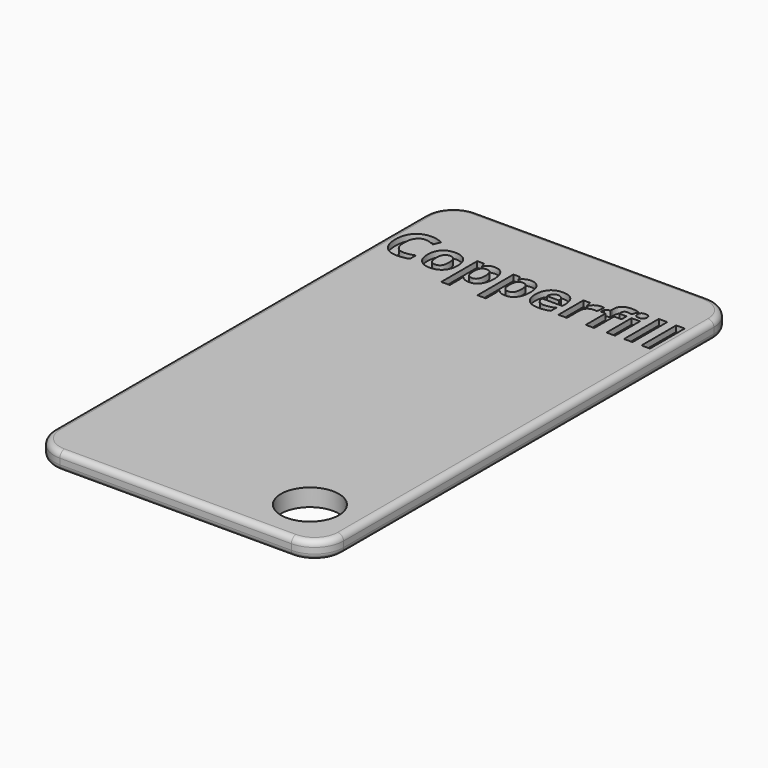
from build123d import *

# Parameters (mm, degrees)
F0_W         = 90
F0_H         = 50
F1_DEPTH     = 3
F2_R         = 1
F3_T1_DEPTH  = 3
F3_T4_ANGLE  = 90
F3_T6_ANGLE  = 90
F3_T8_ANGLE  = 90
F3_T10_ANGLE = 90
F3_T12_ANGLE = 90
F3_T14_ANGLE = 90
F3_T16_ANGLE = 90
F3_T18_ANGLE = 90
F5_ANGLE     = 90
F6_TEXT_SIZE = 9.8841698842
F7_DEPTH     = 1
F8_R         = 5
F9_DEPTH     = 3


# Not quite as in the source:
# - a fillet or chamfer that OpenCascade refuses, or shapes differently, is made with other operations: its cross-section is extruded or revolved along the edge and cut away or added
# - Text() gives the source's letters only with a copy of the font that has no kerning and outlines rounded to 1/6400 em; it was checked with that copy


with BuildPart() as f1:
    # F0 (on Top) → F1 (new body)
    with BuildSketch(Plane.XY):
        Rectangle(F0_W, F0_H)
    extrude(amount=F1_DEPTH)

    # F2
    f2_edges = [f1.edges().sort_by_distance(p)[0] for p in [
        (0, 25, 3),
        (-45, 0, 3),
        (0, -25, 3),
        (45, 0, 3),
        (0, 25, 0),
        (-45, 0, 0),
        (0, -25, 0),
        (45, 0, 0),
    ]]
    fillet(f2_edges, radius=F2_R)

    # F3: fillet of radius 5 on 4 edges, made by hand

    # F3_s2 → F3_t1 (cut)
    with BuildSketch(Plane.XY):
        with BuildLine():
            ThreePointArc((45, -20), (43.5355339059, -23.5355339059), (40, -25))
            Line((40, -25), (45, -25))
            Line((45, -25), (45, -20))
        make_face()
        with BuildLine():
            ThreePointArc((40, 25), (43.5355339059, 23.5355339059), (45, 20))
            Line((45, 20), (45, 25))
            Line((45, 25), (40, 25))
        make_face()
        with BuildLine():
            ThreePointArc((-40, 25), (-43.5355339059, 23.5355339059), (-45, 20))
            Line((-45, 20), (-45, 25))
            Line((-45, 25), (-40, 25))
        make_face()
        with BuildLine():
            ThreePointArc((-45, -20), (-43.5355339059, -23.5355339059), (-40, -25))
            Line((-40, -25), (-45, -25))
            Line((-45, -25), (-45, -20))
        make_face()
    extrude(amount=F3_T1_DEPTH, mode=Mode.SUBTRACT)

    # F3_s3 → F3_t4 (revolve, cut)
    with BuildSketch(Plane.YZ.offset(-40)):
        with BuildLine():
            ThreePointArc((-24, 0), (-24.7071067812, 0.2928932188), (-25, 1))
            Line((-25, 1), (-25, 0))
            Line((-25, 0), (-24, 0))
        make_face()
    revolve(axis=Axis((-40, -20, 0), (0, 0, -1)), revolution_arc=F3_T4_ANGLE, mode=Mode.SUBTRACT)

    # F3_s5 → F3_t6 (revolve, cut)
    with BuildSketch(Plane.XZ.offset(20)):
        with BuildLine():
            ThreePointArc((-44, 3), (-44.7071067812, 2.7071067812), (-45, 2))
            Line((-45, 2), (-45, 3))
            Line((-45, 3), (-44, 3))
        make_face()
    revolve(axis=Axis((-40, -20, 3), (0, 0, 1)), revolution_arc=F3_T6_ANGLE, mode=Mode.SUBTRACT)

    # F3_s7 → F3_t8 (revolve, cut)
    with BuildSketch(Plane.XZ.offset(-20)):
        with BuildLine():
            ThreePointArc((-44, 0), (-44.7071067812, 0.2928932188), (-45, 1))
            Line((-45, 1), (-45, 0))
            Line((-45, 0), (-44, 0))
        make_face()
    revolve(axis=Axis((-40, 20, 0), (0, 0, -1)), revolution_arc=F3_T8_ANGLE, mode=Mode.SUBTRACT)

    # F3_s9 → F3_t10 (revolve, cut)
    with BuildSketch(Plane.YZ.offset(-40)):
        with BuildLine():
            ThreePointArc((24, 3), (24.7071067812, 2.7071067812), (25, 2))
            Line((25, 2), (25, 3))
            Line((25, 3), (24, 3))
        make_face()
    revolve(axis=Axis((-40, 20, 3), (0, 0, 1)), revolution_arc=F3_T10_ANGLE, mode=Mode.SUBTRACT)

    # F3_s11 → F3_t12 (revolve, cut)
    with BuildSketch(Plane.YZ.offset(40)):
        with BuildLine():
            ThreePointArc((24, 0), (24.7071067812, 0.2928932188), (25, 1))
            Line((25, 1), (25, 0))
            Line((25, 0), (24, 0))
        make_face()
    revolve(axis=Axis((40, 20, 0), (0, 0, -1)), revolution_arc=F3_T12_ANGLE, mode=Mode.SUBTRACT)

    # F3_s13 → F3_t14 (revolve, cut)
    with BuildSketch(Plane.XZ.offset(-20)):
        with BuildLine():
            ThreePointArc((44, 3), (44.7071067812, 2.7071067812), (45, 2))
            Line((45, 2), (45, 3))
            Line((45, 3), (44, 3))
        make_face()
    revolve(axis=Axis((40, 20, 3), (0, 0, 1)), revolution_arc=F3_T14_ANGLE, mode=Mode.SUBTRACT)

    # F3_s15 → F3_t16 (revolve, cut)
    with BuildSketch(Plane.XZ.offset(20)):
        with BuildLine():
            ThreePointArc((44, 0), (44.7071067812, 0.2928932188), (45, 1))
            Line((45, 1), (45, 0))
            Line((45, 0), (44, 0))
        make_face()
    revolve(axis=Axis((40, -20, 0), (0, 0, -1)), revolution_arc=F3_T16_ANGLE, mode=Mode.SUBTRACT)

    # F3_s17 → F3_t18 (revolve, cut)
    with BuildSketch(Plane.YZ.offset(40)):
        with BuildLine():
            ThreePointArc((-24, 3), (-24.7071067812, 2.7071067812), (-25, 2))
            Line((-25, 2), (-25, 3))
            Line((-25, 3), (-24, 3))
        make_face()
    revolve(axis=Axis((40, -20, 3), (0, 0, 1)), revolution_arc=F3_T18_ANGLE, mode=Mode.SUBTRACT)


with BuildPart() as f1_1:
    # F5: moved
    add(f1.part.rotate(Axis((0, 0, 16.4477843791), (0, 0, 1)), F5_ANGLE))

    # F6 (on face) → F7 (cut)
    with BuildSketch(Plane.XY.offset(3)):
        with Locations((-24, 28.2511197179)):
            Text('Copperfill', F6_TEXT_SIZE, font='Open Sans', font_style=FontStyle.BOLD, text_align=(TextAlign.LEFT, TextAlign.BOTTOM))
    extrude(amount=-F7_DEPTH, mode=Mode.SUBTRACT)

    # F8 (on face) → F9 (cut)
    with BuildSketch(Plane.XY.offset(3)):
        with Locations((16, -36)):
            Circle(F8_R)
    extrude(amount=-F9_DEPTH, mode=Mode.SUBTRACT)


solid = f1_1.part
